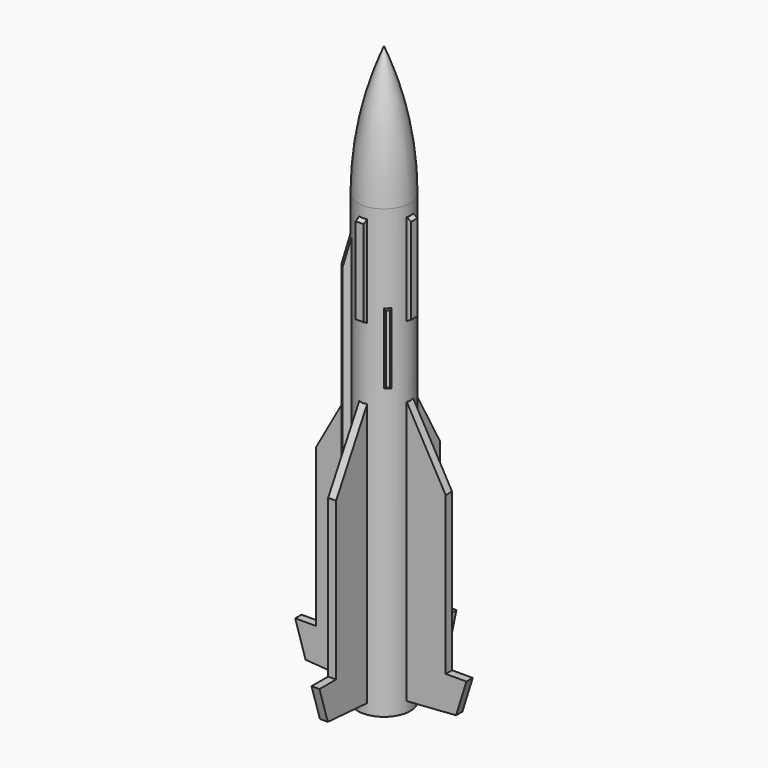
from build123d import *

# Parameters (mm, degrees)
F4_DEPTH      = 0.2
F5_COUNT      = 4
F8_DEPTH      = 16.1805555556
F11_DEPTH     = 3.6111111111
F12_SIZE2     = 0.347212
F12_SIZE      = 1.295841
F13_T4_DEPTH  = 4.1254477087
F13_S5_R      = 1.3194444444
F13_T6_DEPTH  = 4
F13_T10_DEPTH = 4.1254477087
F13_S11_R     = 1.3194444444
F13_T12_DEPTH = 4
F13_T16_DEPTH = 0.8615588198
F13_S17_R     = 1.3194444444
F13_T18_DEPTH = 2
F13_T22_DEPTH = 0.8615588198
F13_S23_R     = 1.3194444444
F13_T24_DEPTH = 2


# Not quite as in the source:
# - a fillet or chamfer that OpenCascade refuses, or shapes differently, is made with other operations: its cross-section is extruded or revolved along the edge and cut away or added
# - a fillet or chamfer is up to 0.001 mm smaller than in the source, because OpenCascade refuses the exact size


with BuildPart() as f2:
    # F1 (on Front) → F2 (revolve)
    with BuildSketch(Plane.XZ):
        with BuildLine():
            Line((0, 29.0277777778), (0, 0))
            Line((0, 0), (1.3194444444, 0))
            Line((1.3194444444, 0), (1.3194444444, 22.5))
            ThreePointArc((1.3194444444, 22.5), (0.9862812817, 25.8298955073), (0, 29.0277777778))
        make_face()
    revolve(axis=Axis((0, 0, 14.5138888889), (0, 0, 1)))

    # F3 (on Front) → F4 (join, symmetric)
    with BuildSketch(Plane.XZ):
        Polygon((0, 22.7062260496), (0, 0.4279147105), (3.7847222222, 0.6944444444), (4.3055555556, 2.3611111111), (3.2638888889, 2.3611111111), (1.3194444444, 2.3611111111), (0.4, 2.3611111111), (0.4, 2.4652777778), (3.2638888889, 2.4652777778), (3.2638888889, 10.2777777778), (0.4, 15.3918650794), (0.4, 16.8302696136), (1.5277777778, 17.4813924172), (1.5277777778, 21.8241631384), align=None)
        Polygon((1.3194444444, 2.3611111111), (3.2638888889, 2.3611111111), (3.2638888889, 2.4652777778), (0.4, 2.4652777778), (0.4, 2.3611111111), align=None)
    extrude(amount=F4_DEPTH, both=True)

    # F5: F2 ×4 about axis
    f5_axis = Axis((0, 0, 0), (0, 0, 1))


with BuildPart() as f2_1:
    add(f2.part)
    for i in range(1, F5_COUNT):
        add(f2.part.rotate(f5_axis, i * 360 / F5_COUNT))

    # F7 (on offset) → F8 (join)
    with BuildSketch(Plane.XY.offset(3.2291666667)):
        with BuildLine():
            Line((-1.0476380246, -0.8021148367), (-1.3012728959, -1.055749708))
            Line((-1.3012728959, -1.055749708), (-1.055749708, -1.3012728959))
            Line((-1.055749708, -1.3012728959), (-0.8021148367, -1.0476380246))
            ThreePointArc((-0.8021148367, -1.0476380246), (-0.9329881141, -0.9329881141), (-1.0476380246, -0.8021148367))
        make_face()
        with BuildLine():
            Line((-0.8559037867, -0.6103805988), (-1.0476380246, -0.8021148367))
            ThreePointArc((-1.0476380246, -0.8021148367), (-0.9329881141, -0.9329881141), (-0.8021148367, -1.0476380246))
            Line((-0.8021148367, -1.0476380246), (-0.6103805988, -0.8559037867))
            Line((-0.6103805988, -0.8559037867), (-0.8559037867, -0.6103805988))
        make_face()
    extrude(amount=F8_DEPTH)

    # F10 (on offset) → F11 (join)
    with BuildSketch(Plane.XY.offset(14.5138888889)):
        Polygon((0.2052949184, 0.0402282695), (-0.0402282695, -0.2052949184), (0.8593311577, -1.1048543456), (1.1048543456, -0.8593311577), align=None)
    extrude(amount=F11_DEPTH)

    # F12 (size 1.2958509749 and 0.3472222222 in the source; OpenCascade refuses exactly that, so slightly less here)
    f12_edges = [f2_1.edges().sort_by_distance(p)[0] for p in [
        (-0.932988, -0.932988, 19.409722),
        (-0.932988, -0.932988, 3.229167),
    ]]
    f12_side = f2_1.faces().sort_by_distance((-1.319444, 0, 0.228074))[0]
    chamfer(f12_edges, length=F12_SIZE, length2=F12_SIZE2, reference=f12_side)

    # F13: chamfer of 0.1 on 4 edges, made by hand


with BuildPart() as f13_tool2:
    # F13_s3 → F13_t4 (new body)
    with BuildSketch(Plane.XY.offset(14.2567205901)):
        Polygon((0.7886204796, -1.0341436675), (0.9300418358, -1.0341436675), (0.8593311577, -1.1048543456), align=None)
    extrude(amount=F13_T4_DEPTH)

    # F13_s5 → F13_t6 (cut, symmetric)
    with BuildSketch(Plane.XY.offset(16.3)):
        Circle(F13_S5_R)
    extrude(amount=F13_T6_DEPTH, both=True, mode=Mode.SUBTRACT)


with BuildPart() as f2_2:
    add(f2_1.part)

    # F13_t1: cut F13_tool2
    add(f13_tool2.part, mode=Mode.SUBTRACT)


with BuildPart() as f13_tool8:
    # F13_s9 → F13_t10 (new body)
    with BuildSketch(Plane.XY.offset(14.2567205901)):
        Polygon((1.0341436675, -0.7886204796), (1.0341436675, -0.9300418358), (1.1048543456, -0.8593311577), align=None)
    extrude(amount=F13_T10_DEPTH)

    # F13_s11 → F13_t12 (cut, symmetric)
    with BuildSketch(Plane.XY.offset(16.3)):
        Circle(F13_S11_R)
    extrude(amount=F13_T12_DEPTH, both=True, mode=Mode.SUBTRACT)


with BuildPart() as f2_3:
    add(f2_2.part)

    # F13_t7: cut F13_tool8
    add(f13_tool8.part, mode=Mode.SUBTRACT)


with BuildPart() as f13_tool14:
    # F13_s15 → F13_t16 (new body)
    with BuildSketch(Plane(origin=(-0.3046070419, -0.3046070419, 0), x_dir=(0, 0, 1), z_dir=(0.7071067812, 0.7071067812, 0))):
        Polygon((14.5138888889, 1.2888888889), (14.6138888889, 1.3888888889), (14.5138888889, 1.3888888889), align=None)
    extrude(amount=F13_T16_DEPTH)

    # F13_s17 → F13_t18 (cut, symmetric)
    with BuildSketch(Plane.XY.offset(14.6)):
        Circle(F13_S17_R)
    extrude(amount=F13_T18_DEPTH, both=True, mode=Mode.SUBTRACT)


with BuildPart() as f2_4:
    add(f2_3.part)

    # F13_t13: cut F13_tool14
    add(f13_tool14.part, mode=Mode.SUBTRACT)


with BuildPart() as f13_tool20:
    # F13_s21 → F13_t22 (new body)
    with BuildSketch(Plane(origin=(-0.3046070419, -0.3046070419, 0), x_dir=(0, 0, 1), z_dir=(0.7071067812, 0.7071067812, 0))):
        Polygon((18.125, 1.2888888889), (18.025, 1.3888888889), (18.125, 1.3888888889), align=None)
    extrude(amount=F13_T22_DEPTH)

    # F13_s23 → F13_t24 (cut, symmetric)
    with BuildSketch(Plane.XY.offset(18.1)):
        Circle(F13_S23_R)
    extrude(amount=F13_T24_DEPTH, both=True, mode=Mode.SUBTRACT)


with BuildPart() as f2_5:
    add(f2_4.part)

    # F13_t19: cut F13_tool20
    add(f13_tool20.part, mode=Mode.SUBTRACT)


solid = f2_5.part
